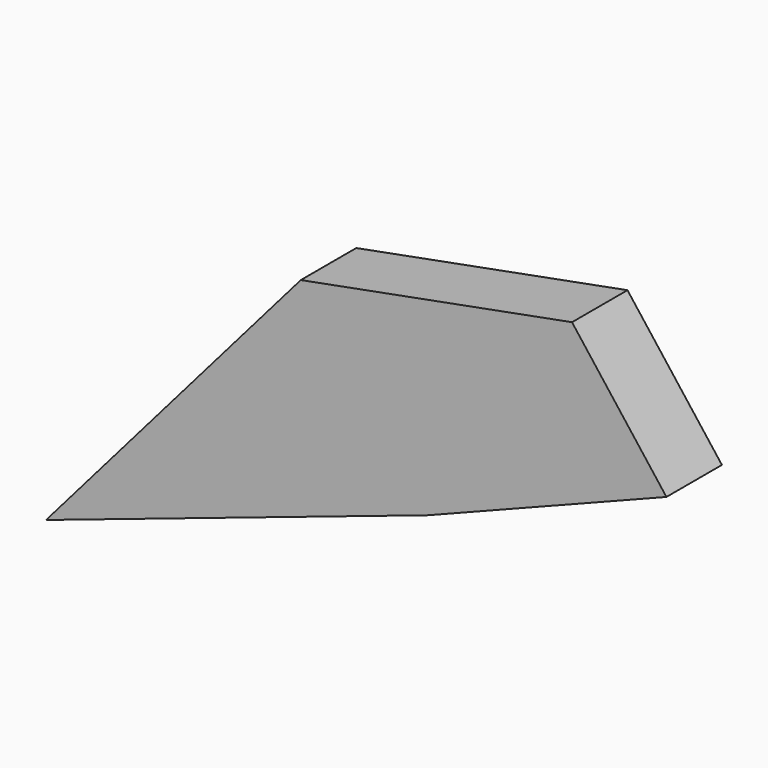
from build123d import *

# Parameters (mm, degrees)
F1_DEPTH = 18.796


# Not quite as in the source:
# - the program builds the solid bodies; features that only make, move or delete a surface that nothing else refers to are left out


with BuildPart() as f1:
    # F0 (on Front) → F1 (new body)
    with BuildSketch(Plane.XZ):
        Polygon((-34.4498695163, 44.9158253761), (0, 0), (64.659229215, 25.390607867), (39.0626974404, 58.7634295225), align=None)
        Polygon((-103.4818813205, -34.7814559937), (0, 0), (-34.4498695163, 44.9158253761), align=None)
    extrude(amount=F1_DEPTH)


solid = f1.part
